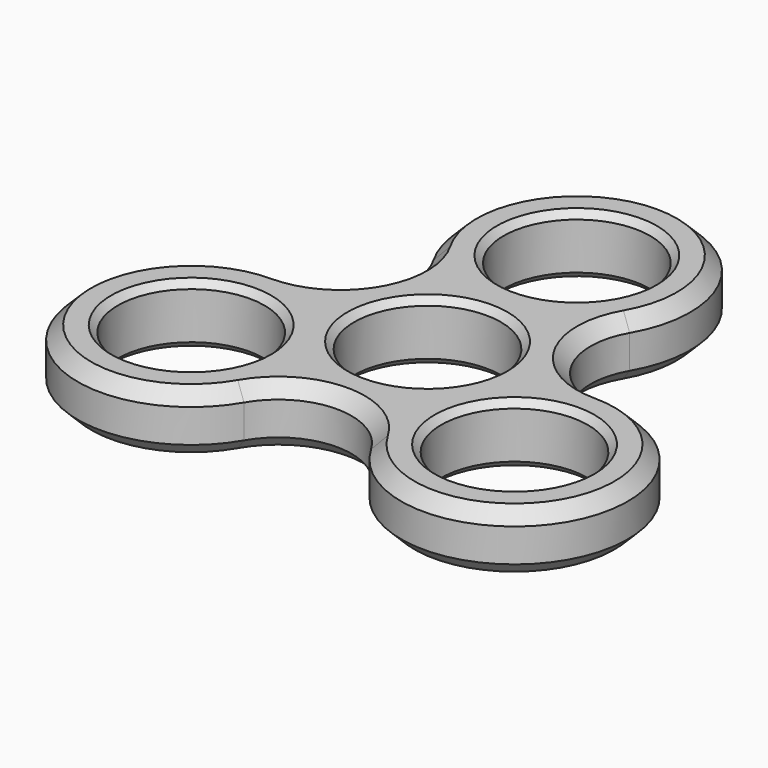
from build123d import *

# Parameters (mm, degrees)
F0_R     = 11
F1_DEPTH = 4.5
F4_SIZE  = 2
F5_SIZE  = 1


# Not quite as in the source:
# - a feature of the source that left no trace in its solid (it failed there, or was rolled back) is left out


with BuildPart() as f1:
    # F0 (on Top) → F1 (new body, symmetric)
    with BuildSketch(Plane.XY):
        with BuildLine():
            ThreePointArc((-24.248711306, 3), (-38.9711431703, -22.5), (-9.5262794416, -22.5))
            ThreePointArc((-9.5262794416, -22.5), (0, -17), (9.5262794416, -22.5))
            ThreePointArc((9.5262794416, -22.5), (38.9711431703, -22.5), (24.248711306, 3))
            ThreePointArc((24.248711306, 3), (14.7224318643, 8.5), (14.7224318643, 19.5))
            ThreePointArc((14.7224318643, 19.5), (0, 45), (-14.7224318643, 19.5))
            ThreePointArc((-14.7224318643, 19.5), (-14.7224318643, 8.5), (-24.248711306, 3))
        make_face()
        with Locations((-24.248711306, -14)):
            Circle(F0_R, mode=Mode.SUBTRACT)
        with Locations((24.248711306, -14)):
            Circle(F0_R, mode=Mode.SUBTRACT)
        Circle(F0_R, mode=Mode.SUBTRACT)
        with Locations((0, 28)):
            Circle(F0_R, mode=Mode.SUBTRACT)
    extrude(amount=F1_DEPTH, both=True)

    # F4
    f4_edges = [f1.edges().sort_by_distance(p)[0] for p in [
        (-38.971143, -22.5, 4.5),
        (-38.971143, -22.5, -4.5),
        (-14.722432, 8.5, -4.5),
        (-14.722432, 8.5, 4.5),
        (0, 45, -4.5),
        (0, 45, 4.5),
        (14.722432, 8.5, -4.5),
        (14.722432, 8.5, 4.5),
        (38.971143, -22.5, -4.5),
        (38.971143, -22.5, 4.5),
        (0, -17, -4.5),
        (0, -17, 4.5),
    ]]
    chamfer(f4_edges, length=F4_SIZE)

    # F5
    f5_edges = [f1.edges().sort_by_distance(p)[0] for p in [
        (-35.248711, -14, 4.5),
        (-13.248711, -14, 0),
        (-35.248711, -14, -4.5),
        (-11, 0, 4.5),
        (11, 0, 0),
        (-11, 0, -4.5),
        (-11, 28, 4.5),
        (11, 28, 0),
        (-11, 28, -4.5),
        (13.248711, -14, 4.5),
        (35.248711, -14, 0),
        (13.248711, -14, -4.5),
    ]]
    chamfer(f5_edges, length=F5_SIZE)


solid = f1.part
